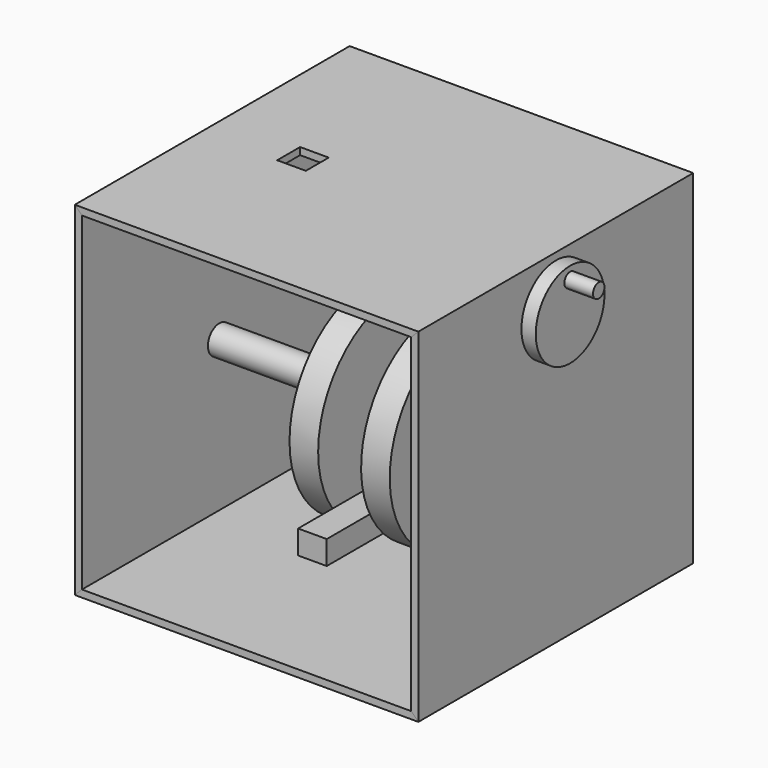
from build123d import *

# Parameters (mm, degrees)
F0_R      = 3.175
F1_DEPTH  = 304.8
F3_R      = 31.75
F4_DEPTH  = 38.1
F6_W      = 304.8
F6_H      = 304.8
F6_W_2    = 25.4
F6_H_2    = 25.4
F7_DEPTH  = 6.35
F8_SIZE   = 6.34999
F9_W      = 304.8
F9_H      = 304.8
F10_DEPTH = 6.35
F11_SIZE  = 6.34999
F13_W     = 304.8
F13_H     = 304.8
F14_DEPTH = 6.35
F15_SIZE  = 6.34999
F17_W     = 304.8
F17_H     = 304.8
F18_DEPTH = 6.35
F19_SIZE  = 6.34999
F22_DEPTH = 25.4
F23_R     = 9.525
F24_DEPTH = 38.1
F26_W     = 304.8
F26_H     = 304.8
F27_DEPTH = 6.35
F28_SIZE  = 6.34999
F29_R     = 38.1
F30_DEPTH = 12.7
F31_R     = 6.35
F32_DEPTH = 25.4
F33_R     = 12.7
F34_DEPTH = 69.85
F36_R     = 88.9
F37_DEPTH = 25.4
F38_R     = 12.7
F39_DEPTH = 134.62
F41_DEPTH = 25.4


# Not quite as in the source:
# - a fillet or chamfer is up to 0.001 mm smaller than in the source, because OpenCascade refuses the exact size
# - a feature of the source that left no trace in its solid (it failed there, or was rolled back) is left out


with BuildPart() as f1:
    # F0 (on Right) → F1 (new body)
    with BuildSketch(Plane.YZ):
        Circle(F0_R)
    extrude(amount=F1_DEPTH)

    # F3 (on offset) → F4 (join)
    with BuildSketch(Plane.YZ.offset(63.5)):
        with Locations((0, -25.4)):
            Circle(F3_R)
    extrude(amount=F4_DEPTH)

    # F21 (on offset) → F22, piece 2 (join)
    with BuildSketch(Plane.YZ.offset(203.2)):
        with BuildLine():
            ThreePointArc((-9.51e-08, -31.75), (22.4506402691, -22.4506403363), (31.75, 0))
            ThreePointArc((31.75, 0), (-22.4506402691, 22.4506403363), (-9.51e-08, -31.75))
        make_face()
    extrude(amount=F22_DEPTH)


with BuildPart() as f7:
    # F6 (on offset) → F7 (new body)
    with BuildSketch(Plane.XY.offset(38.1)):
        with Locations((152.4, 0)):
            Rectangle(F6_W, F6_H)
        with Locations((80.4958567023, 0)):
            Rectangle(F6_W_2, F6_H_2, mode=Mode.SUBTRACT)
    extrude(amount=F7_DEPTH)

    # F8 (size 6.35 in the source; OpenCascade refuses exactly that, so slightly less here)
    f8_edges = [f7.edges().sort_by_distance(p)[0] for p in [
        (304.8, 0, 38.1),
        (152.4, 152.4, 38.1),
        (0, 0, 38.1),
    ]]
    chamfer(f8_edges, length=F8_SIZE)


with BuildPart() as f10:
    # F9 (on Right) → F10 (new body)
    with BuildSketch(Plane.YZ):
        with Locations((0, -107.95)):
            Rectangle(F9_W, F9_H)
    extrude(amount=F10_DEPTH)

    # F11 (size 6.35 in the source; OpenCascade refuses exactly that, so slightly less here)
    f11_edges = [f10.edges().sort_by_distance(p)[0] for p in [
        (6.35, 0, 44.45),
        (6.35, 0, -260.35),
        (6.35, 152.4, -107.95),
    ]]
    chamfer(f11_edges, length=F11_SIZE)


with BuildPart() as f14:
    # F13 (on offset) → F14 (new body)
    with BuildSketch(Plane.XZ.offset(-152.4)):
        with Locations((152.4, -107.95)):
            Rectangle(F13_W, F13_H)
    extrude(amount=F14_DEPTH)

    # F15 (size 6.35 in the source; OpenCascade refuses exactly that, so slightly less here)
    f15_edges = [f14.edges().sort_by_distance(p)[0] for p in [
        (152.4, 146.05, 44.45),
        (304.8, 146.05, -107.95),
        (152.4, 146.05, -260.35),
        (0, 146.05, -107.95),
    ]]
    chamfer(f15_edges, length=F15_SIZE)


with BuildPart() as f18:
    # F17 (on offset) → F18 (new body)
    with BuildSketch(Plane.XY.offset(-260.35)):
        with Locations((152.4, 0)):
            Rectangle(F17_W, F17_H)
    extrude(amount=F18_DEPTH)

    # F19 (size 6.35 in the source; OpenCascade refuses exactly that, so slightly less here)
    f19_edges = [f18.edges().sort_by_distance(p)[0] for p in [
        (0, 0, -254),
        (152.4, 152.4, -254),
        (304.8, 0, -254),
    ]]
    chamfer(f19_edges, length=F19_SIZE)


with BuildPart() as f22:
    # F21 (on offset) → F22 (new body)
    with BuildSketch(Plane.YZ.offset(203.2)):
        with BuildLine():
            ThreePointArc((88.9, -120.65), (62.8617928139, -57.7882071189), (-9.51e-08, -31.75))
            ThreePointArc((-9.51e-08, -31.75), (-62.8617928139, -183.5117928811), (88.9, -120.65))
        make_face()
    extrude(amount=F22_DEPTH)


with BuildPart() as f24:
    # F23 (on face) → F24 (new body)
    with BuildSketch(Plane(origin=(203.2, 0, 0), x_dir=(0, -1, 0), z_dir=(-1, 0, 0))):
        with Locations((0, -171.45)):
            Circle(F23_R)
    extrude(amount=F24_DEPTH)

    # F36 (on offset) → F37 (join)
    with BuildSketch(Plane(origin=(165.1, 0, 0), x_dir=(0, -1, 0), z_dir=(-1, 0, 0))):
        with Locations((0, -120.65)):
            Circle(F36_R)
    extrude(amount=F37_DEPTH)


with BuildPart() as f27:
    # F26 (on offset) → F27 (new body)
    with BuildSketch(Plane.YZ.offset(304.8)):
        with Locations((0, -107.95)):
            Rectangle(F26_W, F26_H)
    extrude(amount=-F27_DEPTH)

    # F28 (size 6.35 in the source; OpenCascade refuses exactly that, so slightly less here)
    f28_edges = [f27.edges().sort_by_distance(p)[0] for p in [
        (298.45, 0, 44.45),
        (298.45, 152.4, -107.95),
        (298.45, 0, -260.35),
    ]]
    chamfer(f28_edges, length=F28_SIZE)


with BuildPart() as f30:
    # F29 (on face) → F30 (new body)
    with BuildSketch(Plane.YZ.offset(304.8)):
        Circle(F29_R)
    extrude(amount=F30_DEPTH)

    # F31 (on face) → F32 (join)
    with BuildSketch(Plane.YZ.offset(317.5)):
        with Locations((0, 27.0901415497)):
            Circle(F31_R)
    extrude(amount=F32_DEPTH)


with BuildPart() as f34:
    # F33 (on face) → F34 (new body)
    with BuildSketch(Plane.YZ.offset(228.6)):
        with Locations((0, -120.65)):
            Circle(F33_R)
    extrude(amount=F34_DEPTH)


with BuildPart() as f39:
    # F38 (on face) → F39 (new body)
    with BuildSketch(Plane(origin=(139.7, 0, 0), x_dir=(0, -1, 0), z_dir=(-1, 0, 0))):
        with Locations((0, -120.65)):
            Circle(F38_R)
    extrude(amount=F39_DEPTH)


with BuildPart() as f41:
    # F40 (on face) → F41 (new body)
    with BuildSketch(Plane.YZ.offset(203.2)):
        with BuildLine():
            ThreePointArc((-15.8678864062, -181.991), (-19.05, -171.45), (-15.8678864062, -160.909))
            Line((-15.8678864062, -160.909), (-127, -160.909))
            Line((-127, -160.909), (-127, -181.991))
            Line((-127, -181.991), (-15.8678864062, -181.991))
        make_face()
        with BuildLine():
            Line((0, -160.909), (-15.8678864062, -160.909))
            ThreePointArc((-15.8678864062, -160.909), (-19.05, -171.45), (-15.8678864062, -181.991))
            Line((-15.8678864062, -181.991), (0, -181.991))
            ThreePointArc((0, -181.991), (-10.541, -171.45), (0, -160.909))
        make_face()
        with BuildLine():
            ThreePointArc((-15.8678864062, -181.991), (5.5054184202, -189.6871288316), (19.05, -171.45))
            ThreePointArc((19.05, -171.45), (5.5054184202, -153.2128711684), (-15.8678864062, -160.909))
            Line((-15.8678864062, -160.909), (0, -160.909))
            ThreePointArc((0, -160.909), (7.4536125805, -163.9963874195), (10.541, -171.45))
            ThreePointArc((10.541, -171.45), (7.4536125805, -178.9036125805), (0, -181.991))
            Line((0, -181.991), (-15.8678864062, -181.991))
        make_face()
    extrude(amount=-F41_DEPTH)


solid = Compound([f1.part, f7.part, f10.part, f14.part, f18.part, f22.part, f24.part, f27.part, f30.part, f34.part, f39.part, f41.part])
